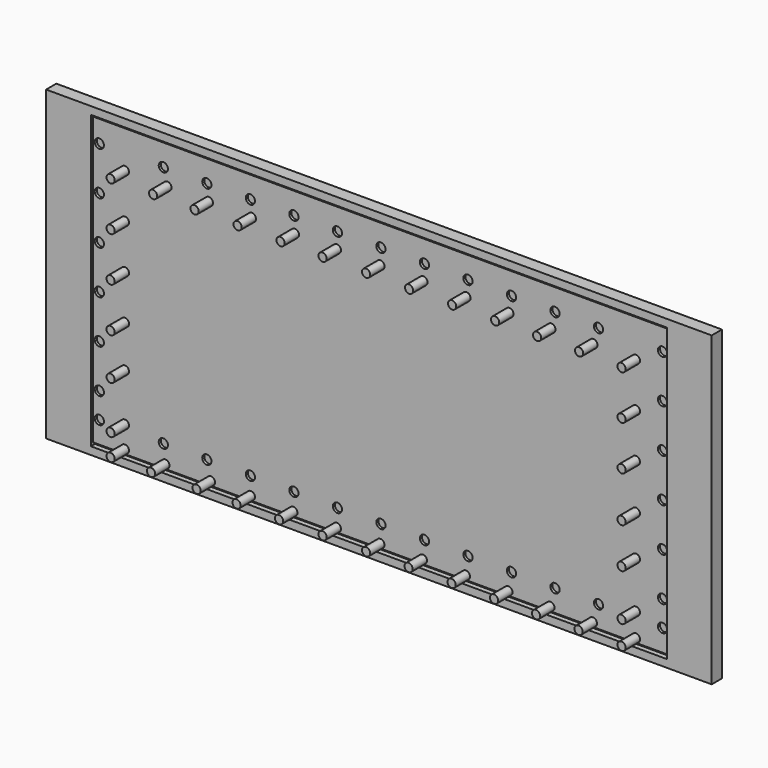
from build123d import *

# Parameters (mm, degrees)
F0_W     = 1200
F0_H     = 560
F0_R     = 9
F1_DEPTH = 20
F2_W     = 1300
F2_H     = 600
F2_W_2   = 900
F2_H_2   = 365
F3_DEPTH = 25
F4_W     = 1125
F4_H     = 570
F4_W_2   = 900
F4_H_2   = 365
F5_DEPTH = 10
F6_R     = 8
F7_DEPTH = 40


with BuildPart() as f1:
    # F0 (on Front) → F1 (new body)
    with BuildSketch(Plane.XZ):
        Rectangle(F0_W, F0_H)
        with Locations((-550, -237.5)):
            Circle(F0_R, mode=Mode.SUBTRACT)
        with Locations((-425, -237.5)):
            Circle(F0_R, mode=Mode.SUBTRACT)
        with Locations((-340, -237.5)):
            Circle(F0_R, mode=Mode.SUBTRACT)
        with Locations((-550, -187.5)):
            Circle(F0_R, mode=Mode.SUBTRACT)
        with Locations((-255, -237.5)):
            Circle(F0_R, mode=Mode.SUBTRACT)
        with Locations((-170, -237.5)):
            Circle(F0_R, mode=Mode.SUBTRACT)
        with Locations((-85, -237.5)):
            Circle(F0_R, mode=Mode.SUBTRACT)
        with Locations((-550, -102.5)):
            Circle(F0_R, mode=Mode.SUBTRACT)
        with Locations((-550, -17.5)):
            Circle(F0_R, mode=Mode.SUBTRACT)
        with Locations((0, -237.5)):
            Circle(F0_R, mode=Mode.SUBTRACT)
        with Locations((85, -237.5)):
            Circle(F0_R, mode=Mode.SUBTRACT)
        with Locations((170, -237.5)):
            Circle(F0_R, mode=Mode.SUBTRACT)
        with Locations((255, -237.5)):
            Circle(F0_R, mode=Mode.SUBTRACT)
        with Locations((340, -237.5)):
            Circle(F0_R, mode=Mode.SUBTRACT)
        with Locations((425, -237.5)):
            Circle(F0_R, mode=Mode.SUBTRACT)
        with Locations((550, -237.5)):
            Circle(F0_R, mode=Mode.SUBTRACT)
        with Locations((550, -187.5)):
            Circle(F0_R, mode=Mode.SUBTRACT)
        with Locations((550, -102.5)):
            Circle(F0_R, mode=Mode.SUBTRACT)
        with Locations((550, -17.5)):
            Circle(F0_R, mode=Mode.SUBTRACT)
        with Locations((-550, 67.5)):
            Circle(F0_R, mode=Mode.SUBTRACT)
        with Locations((-550, 152.5)):
            Circle(F0_R, mode=Mode.SUBTRACT)
        with Locations((-550, 237.5)):
            Circle(F0_R, mode=Mode.SUBTRACT)
        with Locations((-425, 237.5)):
            Circle(F0_R, mode=Mode.SUBTRACT)
        with Locations((-340, 237.5)):
            Circle(F0_R, mode=Mode.SUBTRACT)
        with Locations((-255, 237.5)):
            Circle(F0_R, mode=Mode.SUBTRACT)
        with Locations((-170, 237.5)):
            Circle(F0_R, mode=Mode.SUBTRACT)
        with Locations((-85, 237.5)):
            Circle(F0_R, mode=Mode.SUBTRACT)
        with Locations((550, 67.5)):
            Circle(F0_R, mode=Mode.SUBTRACT)
        with Locations((0, 237.5)):
            Circle(F0_R, mode=Mode.SUBTRACT)
        with Locations((85, 237.5)):
            Circle(F0_R, mode=Mode.SUBTRACT)
        with Locations((170, 237.5)):
            Circle(F0_R, mode=Mode.SUBTRACT)
        with Locations((255, 237.5)):
            Circle(F0_R, mode=Mode.SUBTRACT)
        with Locations((550, 152.5)):
            Circle(F0_R, mode=Mode.SUBTRACT)
        with Locations((340, 237.5)):
            Circle(F0_R, mode=Mode.SUBTRACT)
        with Locations((425, 237.5)):
            Circle(F0_R, mode=Mode.SUBTRACT)
        with Locations((550, 237.5)):
            Circle(F0_R, mode=Mode.SUBTRACT)
    extrude(amount=F1_DEPTH)


with BuildPart() as f3:
    # F2 (on Front) → F3 (new body)
    with BuildSketch(Plane.XZ):
        Rectangle(F2_W, F2_H)
        with Locations((0, -25)):
            Rectangle(F2_W_2, F2_H_2, mode=Mode.SUBTRACT)
    extrude(amount=F3_DEPTH)

    # F4 (on face) → F5 (cut)
    with BuildSketch(Plane.XZ.offset(25)):
        Rectangle(F4_W, F4_H)
        with Locations((0, -25)):
            Rectangle(F4_W_2, F4_H_2, mode=Mode.SUBTRACT)
    extrude(amount=-F5_DEPTH, mode=Mode.SUBTRACT)

    # F6 (on face) → F7 (join)
    with BuildSketch(Plane.XZ.offset(15)):
        with Locations((-500, 207.5)):
            Circle(F6_R)
        with Locations((-500, 120.5)):
            Circle(F6_R)
        with Locations((-500, 33.5)):
            Circle(F6_R)
        with Locations((-500, -53.5)):
            Circle(F6_R)
        with Locations((-500, -135.5)):
            Circle(F6_R)
        with Locations((-500, -228.5)):
            Circle(F6_R)
        with Locations((-500, -271.5)):
            Circle(F6_R)
        with Locations((-421, -271.5)):
            Circle(F6_R)
        with Locations((-332, -271.5)):
            Circle(F6_R)
        with Locations((-254, -271.5)):
            Circle(F6_R)
        with Locations((-171, -271.5)):
            Circle(F6_R)
        with Locations((-86, -271.5)):
            Circle(F6_R)
        with Locations((-1, -271.5)):
            Circle(F6_R)
        with Locations((82, -271.5)):
            Circle(F6_R)
        with Locations((166, -271.5)):
            Circle(F6_R)
        with Locations((249, -271.5)):
            Circle(F6_R)
        with Locations((414, -271.5)):
            Circle(F6_R)
        with Locations((498, -271.5)):
            Circle(F6_R)
        with Locations((331, -271.5)):
            Circle(F6_R)
        with Locations((498, -225.5)):
            Circle(F6_R)
        with Locations((498, -134.5)):
            Circle(F6_R)
        with Locations((498, -55.5)):
            Circle(F6_R)
        with Locations((498, 33.5)):
            Circle(F6_R)
        with Locations((498, 120.5)):
            Circle(F6_R)
        with Locations((498, 207.5)):
            Circle(F6_R)
        with Locations((415, 207.5)):
            Circle(F6_R)
        with Locations((333, 207.5)):
            Circle(F6_R)
        with Locations((251, 207.5)):
            Circle(F6_R)
        with Locations((167, 207.5)):
            Circle(F6_R)
        with Locations((83, 207.5)):
            Circle(F6_R)
        with Locations((-1, 207.5)):
            Circle(F6_R)
        with Locations((-86, 207.5)):
            Circle(F6_R)
        with Locations((-168, 207.5)):
            Circle(F6_R)
        with Locations((-252, 207.5)):
            Circle(F6_R)
        with Locations((-336, 207.5)):
            Circle(F6_R)
        with Locations((-417, 207.5)):
            Circle(F6_R)
    extrude(amount=F7_DEPTH)


solid = Compound([f1.part, f3.part])
